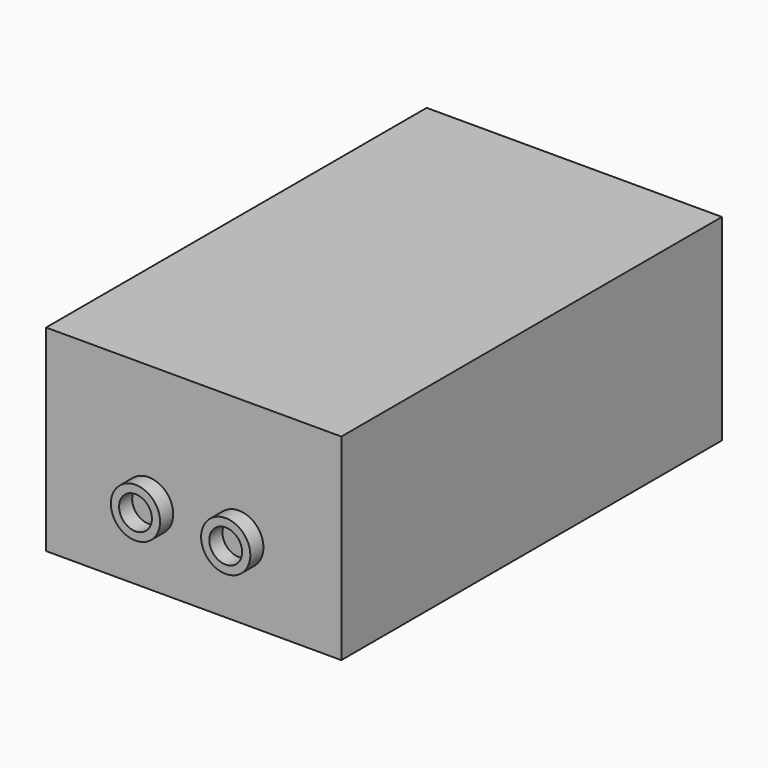
from build123d import *

# Parameters (mm, degrees)
F1_DEPTH = 152.4
F2_DEPTH = 31.75
F3_W     = 73.3992542744
F3_H     = 43.9409847975
F3_W_2   = 60.6992542744
F3_H_2   = 31.2409847975
F4_DEPTH = 6.35
F5_SIZE  = 2.54
F6_R     = 19.05
F6_R_2   = 12.7
F7_DEPTH = 12.7


# Not quite as in the source:
# - a feature names something its author has since deleted; it is built from what else it names


with BuildPart() as f1:
    # F0 (on Top) → F1 (new body)
    with BuildSketch(Plane.XY):
        with BuildLine():
            Line((0, 228.6), (0, 44.45))
            ThreePointArc((0, 44.45), (31.4308964237, 31.4308964237), (44.45, 0))
            ThreePointArc((44.45, 0), (31.4308964237, -31.4308964237), (0, -44.45))
            Line((0, -44.45), (0, -139.7))
            Line((0, -139.7), (114.3, -139.7))
            Line((114.3, -139.7), (114.3, 228.6))
            Line((114.3, 228.6), (0, 228.6))
        make_face()
        with BuildLine():
            ThreePointArc((0, -44.45), (-44.45, 0), (0, 44.45))
            Line((0, 44.45), (0, 228.6))
            Line((0, 228.6), (-114.3, 228.6))
            Line((-114.3, 228.6), (-114.3, -139.7))
            Line((-114.3, -139.7), (0, -139.7))
            Line((0, -139.7), (0, -44.45))
        make_face()
        with BuildLine():
            Line((0, 44.45), (0, 0))
            Line((0, 0), (0, -44.45))
            ThreePointArc((0, -44.45), (31.4308964237, -31.4308964237), (44.45, 0))
            ThreePointArc((44.45, 0), (31.4308964237, 31.4308964237), (0, 44.45))
        make_face()
        with BuildLine():
            Line((0, -44.45), (0, 0))
            Line((0, 0), (0, 44.45))
            ThreePointArc((0, 44.45), (-44.45, 0), (0, -44.45))
        make_face()
    extrude(amount=F1_DEPTH)

    # F0 (on Top) → F2 (join)
    with BuildSketch(Plane.XY):
        with BuildLine():
            Line((0, 44.45), (0, 0))
            Line((0, 0), (0, -44.45))
            ThreePointArc((0, -44.45), (31.4308964237, -31.4308964237), (44.45, 0))
            ThreePointArc((44.45, 0), (31.4308964237, 31.4308964237), (0, 44.45))
        make_face()
        with BuildLine():
            Line((0, -44.45), (0, 0))
            Line((0, 0), (0, 44.45))
            ThreePointArc((0, 44.45), (-44.45, 0), (0, -44.45))
        make_face()
    extrude(amount=-F2_DEPTH)

    # F3 (on face) → F4 (join)
    with BuildSketch(Plane(origin=(0, 228.6, 0), x_dir=(-1, 0, 0), z_dir=(0, 1, 0))):
        with Locations((58.9650124311, 110.7811406255)):
            Rectangle(F3_W, F3_H)
        with Locations((58.9650124311, 110.7811406255)):
            Rectangle(F3_W_2, F3_H_2, mode=Mode.SUBTRACT)
    extrude(amount=F4_DEPTH)

    # F5
    f5_edges = [f1.edges().sort_by_distance(p)[0] for p in [
        (-95.66464, 234.95, 110.781141),
        (-58.965012, 234.95, 88.810648),
        (-22.265385, 234.95, 110.781141),
        (-58.965012, 234.95, 132.751633),
    ]]
    chamfer(f5_edges, length=F5_SIZE)

    # F6 (on face) → F7 (join)
    with BuildSketch(Plane.XZ.offset(139.7)):
        with BuildLine():
            ThreePointArc((53.975, 57.15), (34.925, 76.2), (15.875, 57.15))
            ThreePointArc((15.875, 57.15), (34.925, 38.1), (53.975, 57.15))
        make_face()
        with BuildLine():
            ThreePointArc((47.625, 57.15), (34.925, 44.45), (22.225, 57.15))
            ThreePointArc((22.225, 57.15), (34.925, 69.85), (47.625, 57.15))
        make_face(mode=Mode.SUBTRACT)
        with Locations((-34.925, 57.15)):
            Circle(F6_R)
        with Locations((-34.925, 57.15)):
            Circle(F6_R_2, mode=Mode.SUBTRACT)
    extrude(amount=F7_DEPTH)


solid = f1.part
